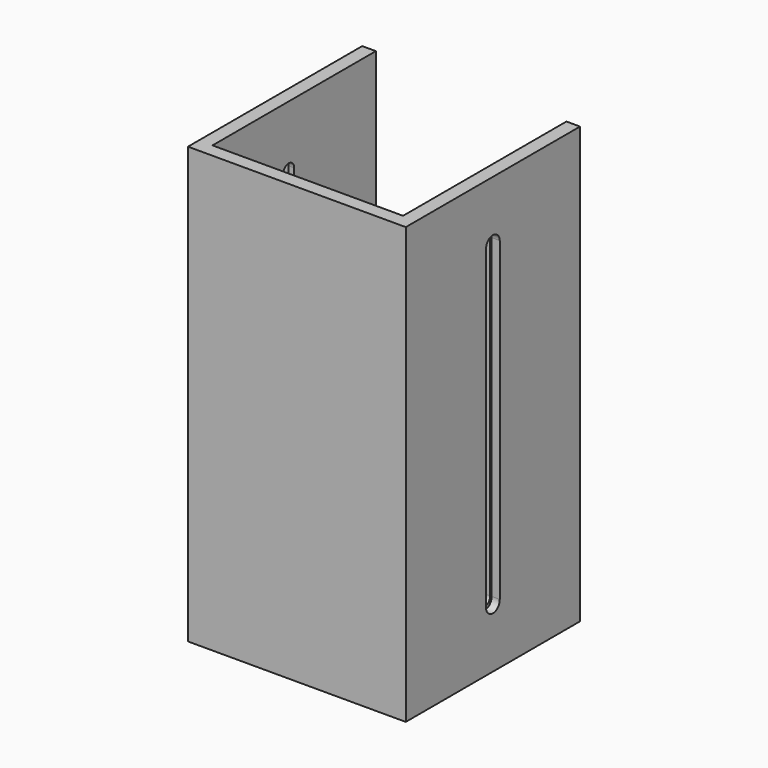
from build123d import *

# Parameters (mm, degrees)
F1_DEPTH      = 101.6
F3_DEPTH      = 287
F3_DEPTH_BACK = 50.801
F5_DEPTH      = 3.81


# Not quite as in the source:
# - an extrude ends at something that could not be found from the text; its depth is read off the source's solid


with BuildPart() as f1:
    # F0 (on Top) → F1 (new body, symmetric)
    with BuildSketch(Plane.XY):
        Polygon((44.45, 101.6), (44.45, 6.35), (0, 6.35), (0, 0), (50.8, 0), (50.8, 101.6), align=None)
    extrude(amount=F1_DEPTH, both=True)

    # F2 (on Right) → F3 (cut, two sides)
    with BuildSketch(Plane.YZ) as f3_sk:
        with BuildLine():
            ThreePointArc((47.625, -73.025), (48.5549359697, -75.2700640303), (50.8, -76.2))
            ThreePointArc((50.8, -76.2), (53.0450640303, -75.2700640303), (53.975, -73.025))
            Line((53.975, -73.025), (53.975, 73.0249999165))
            ThreePointArc((53.975, 73.0249999165), (53.0450640598, 75.2700640008), (50.8, 76.2))
            ThreePointArc((50.8, 76.2), (48.5549359697, 75.2700640303), (47.625, 73.025))
            Line((47.625, 73.025), (47.625, -73.025))
        make_face()
    extrude(amount=-F3_DEPTH, mode=Mode.SUBTRACT)
    extrude(f3_sk.sketch, amount=F3_DEPTH_BACK, mode=Mode.SUBTRACT)

    # F4 (on face) → F5 (cut)
    with BuildSketch(Plane.YZ.offset(50.8)):
        with BuildLine():
            Line((54.7984857559, -73.5657372472), (54.7984857559, 73.7838448219))
            ThreePointArc((54.7984857559, 73.7838448219), (50.7384735742, 77.6595205582), (46.8004034081, 73.66))
            Line((46.8004034081, 73.66), (46.8004034081, -73.740335956))
            ThreePointArc((46.8004034081, -73.740335956), (50.8868960802, -77.6590472365), (54.7984857559, -73.5657372472))
        make_face()
    extrude(amount=-F5_DEPTH, mode=Mode.SUBTRACT)

    # F6: F1 across plane


with BuildPart() as f1_1:
    add(f1.part)
    add(f1.part.mirror(Plane.YZ))


solid = f1_1.part
